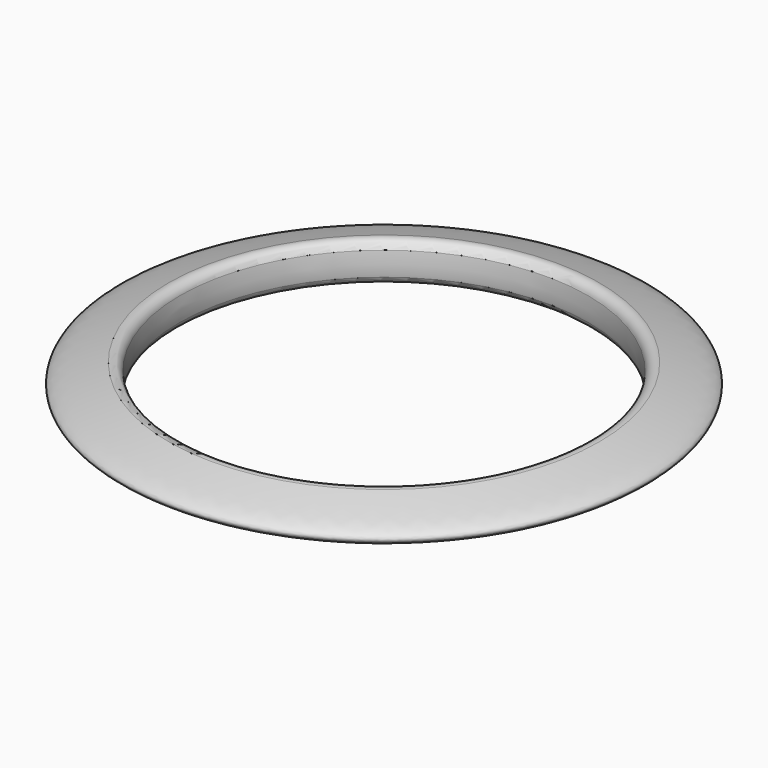
from build123d import *


with BuildPart() as f2:
    # F1 (on Front) → F2 (revolve)
    with BuildSketch(Plane.XZ):
        with BuildLine():
            ThreePointArc((-66.1694296572, 3.789952672), (-67.4877952478, 5.8189480082), (-69.8748672823, 6.2149240268))
            add(Edge.make_bspline(
                [(-69.8748672823, 6.2149240268), (-79.6476224624, 3.7120960185), (-91.7985698992, 0.2172583079), (-79.2830328431, -4.0982824608), (-69.9725030476, -6.3181628118)],
                knots=[0.0461378742, 0.0461378742, 0.0461378742, 0.0461378742, 0.5013801316, 0.9538145198, 0.9538145198, 0.9538145198, 0.9538145198], degree=3))
            ThreePointArc((-69.9725030476, -6.3181628118), (-67.6613636276, -5.9279270401), (-66.3362500715, -3.9946077598))
            add(Edge.make_bspline(
                [(-66.1694296572, 3.789952672), (-65.9639875018, 2.5258200721), (-65.6878006976, -0.0717621899), (-66.0671549323, -2.663953057), (-66.3362500715, -3.9946077598)],
                knots=[0.2288912147, 0.2288912147, 0.2288912147, 0.2288912147, 0.4993772734, 0.7849522853, 0.7849522853, 0.7849522853, 0.7849522853], degree=3))
        make_face()
    revolve(axis=Axis((0, 0, -3.5660378635), (0, 0, -1)))


solid = f2.part
